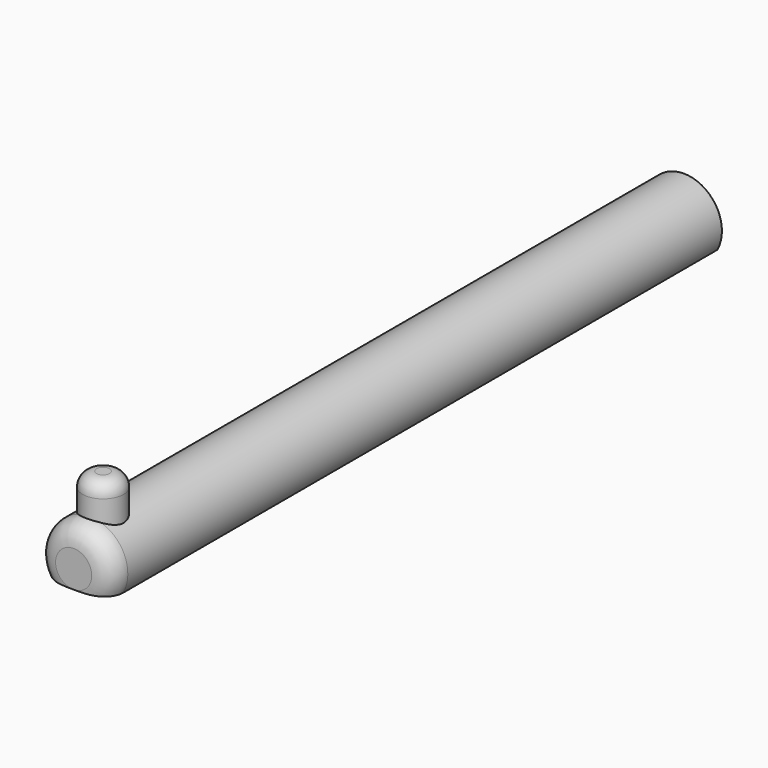
from build123d import *

# Parameters (mm, degrees)
F1_DEPTH    = 150
F2_R        = 4.0142469295
F3_DEPTH    = 14
F4_T4_ANGLE = 359.64
F4_S5_R     = 4.0142469295
F4_T6_DEPTH = 8385
F5_R        = 2.7280613255


# Not quite as in the source:
# - a fillet or chamfer that OpenCascade refuses, or shapes differently, is made with other operations: its cross-section is extruded or revolved along the edge and cut away or added


with BuildPart() as f1:
    # F0 (on Front) → F1 (new body)
    with BuildSketch(Plane.XZ):
        with BuildLine():
            Line((-6.5942404738, -3.5729529208), (6.5942404738, -3.5729529208))
            ThreePointArc((6.5942404738, -3.5729529208), (0, 7.5), (-6.5942404738, -3.5729529208))
        make_face()
    extrude(amount=F1_DEPTH)

    # F2 (on Top) → F3 (join)
    with BuildSketch(Plane.XY):
        with Locations((0, -142.7590548992)):
            Circle(F2_R)
    extrude(amount=F3_DEPTH)

    # F4: fillet of radius 4 on 1 edges, made by hand


with BuildPart() as f4_tool2:
    # F4_s3 → F4_t4 (revolve)
    with BuildSketch(Plane(origin=(0, 0, 0), x_dir=(0, 1, 0), z_dir=(-0.9999950652, 0, -0.0031415875))):
        with BuildLine():
            ThreePointArc((-145.9990343146, 7.5004), (-148.8284271247, 6.3284271247), (-150.0004, 3.4990343146))
            Line((-150.0004, 3.4990343146), (-150.4005365685, 3.4990343146))
            ThreePointArc((-150.4005365685, 3.4990343146), (-150.4001365685, 5.4995171573), (-150.4001365685, 7.5))
            Line((-150.4001365685, 7.5), (-150, 7.9001365685))
            ThreePointArc((-150, 7.9001365685), (-147.9995171573, 7.9001365685), (-145.9990343146, 7.9005365685))
            Line((-145.9990343146, 7.9005365685), (-145.9990343146, 7.5004))
        make_face()
    revolve(axis=Axis((0, -150, 0), (0, -1, 0)), revolution_arc=F4_T4_ANGLE)

    # F4_s5 → F4_t6 (cut, symmetric)
    with BuildSketch(Plane.XY):
        with Locations((0, -142.7590548992)):
            Circle(F4_S5_R)
    extrude(amount=F4_T6_DEPTH, both=True, mode=Mode.SUBTRACT)


with BuildPart() as f1_1:
    add(f1.part)

    # F4_t1: cut F4_tool2
    add(f4_tool2.part, mode=Mode.SUBTRACT)

    # F5
    f5_edges = [f1_1.edges().sort_by_distance(p)[0] for p in [
        (-4.014247, -142.759055, 14),
    ]]
    fillet(f5_edges, radius=F5_R)


solid = f1_1.part
